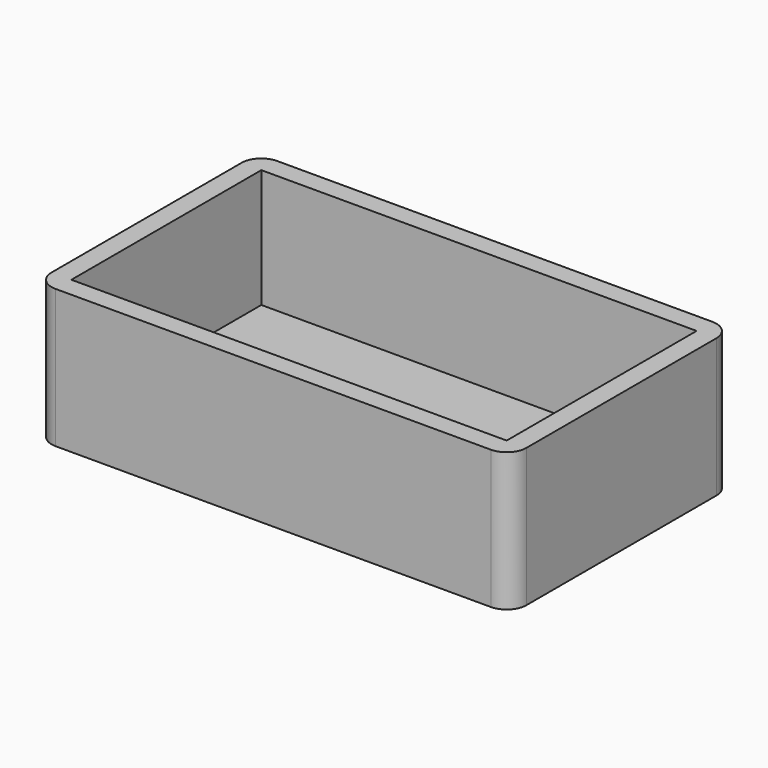
from build123d import *

# Parameters (mm, degrees)
F1_DEPTH = 35
F2_T     = 5


# Not quite as in the source:
# - a shell that OpenCascade refuses in one call is made with other operations: the cavity is built on its own and cut out


with BuildPart() as f1:
    # F0 (on Top) → F1 (new body)
    with BuildSketch(Plane.XY):
        with BuildLine():
            Line((55, 35), (-55, 35))
            ThreePointArc((-55, 35), (-58.5355339059, 33.5355339059), (-60, 30))
            Line((-60, 30), (-60, -30))
            ThreePointArc((-60, -30), (-58.5355339059, -33.5355339059), (-55, -35))
            Line((-55, -35), (55, -35))
            ThreePointArc((55, -35), (58.5355339059, -33.5355339059), (60, -30))
            Line((60, -30), (60, 30))
            ThreePointArc((60, 30), (58.5355339059, 33.5355339059), (55, 35))
        make_face()
    extrude(amount=F1_DEPTH)

    # F2: shell of thickness 5, made by hand


with BuildPart() as f2_core1:
    # F2_t2: copy of F1
    add(f1.part)

    # the walls: a layer under each face that stays
    f2_faces = [f2_core1.faces().sort_by_distance(p)[0] for p in [
        (0, 35, 17.5),
        (-60, 0, 17.5),
        (0, -35, 17.5),
        (60, 0, 17.5),
        (0, 0, 0),
    ]]
    thicken(f2_faces, amount=-F2_T, mode=Mode.SUBTRACT)


with BuildPart() as f1_1:
    add(f1.part)

    # what is left inside the walls is the cavity
    f2_cavity = [f2_core1.part.solids().sort_by_distance(p)[0] for p in [
        (0, -10, 5.05),
    ]]
    add(f2_cavity, mode=Mode.SUBTRACT)


solid = f1_1.part
